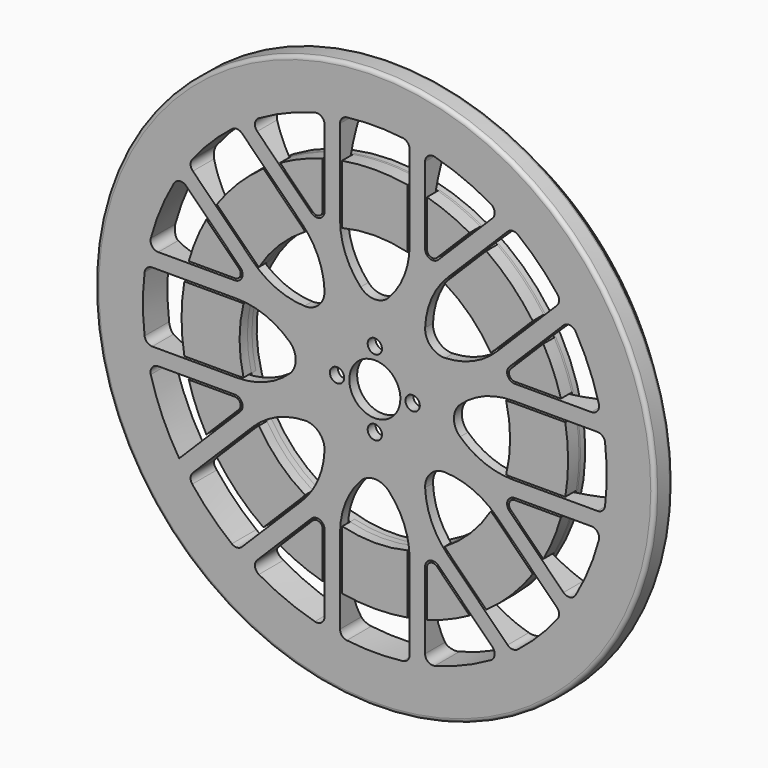
from build123d import *
from build123d import SkipClean  # not in build123d's __all__

# Parameters (mm, degrees)
F3_D      = 3.7
F4_R      = 71
F4_R_2    = 66
F4_R_3    = 6.604
F5_DEPTH  = 13.001
F6_R      = 20
F7_R      = 5
F8_R      = 2
F9_R      = 0.6
F13_DEPTH = 4
F14_R     = 72.39
F14_R_2   = 66
F15_DEPTH = 5.842
F16_R     = 1


with BuildPart() as f1:
    # F0 (on Right) → F1 (revolve)
    with BuildSketch(Plane.YZ):
        with BuildLine():
            Line((0, 66), (0, 6.604))
            Line((0, 6.604), (2.54, 6.604))
            Line((2.54, 6.604), (2.54, 42))
            ThreePointArc((2.54, 42), (5.2686233007, 55.0901833448), (13, 66))
            Line((13, 66), (0, 66))
        make_face()
    revolve(axis=Axis((0, 6.5, 0), (0, 1, 0)))

    # F3 (through all)
    with Locations(Plane.XZ):
        with Locations((0, 9.779), (9.779, 0), (0, -9.779), (-9.779, 0)):
            Hole(F3_D / 2)

    # F4 (on face) → F5 (cut, through all)
    with BuildSketch(Plane.XZ):
        Circle(F4_R)
        Circle(F4_R_2, mode=Mode.SUBTRACT)
        Circle(F4_R_3)
        with BuildLine():
            Line((-13, 25.7279220614), (-35.5824333316, 48.310355393))
            ThreePointArc((-35.5824333316, 48.310355393), (-42.4264068712, 42.4264068712), (-48.310355393, 35.5824333316))
            Line((-48.310355393, 35.5824333316), (-25.7279220614, 13))
            Line((-25.7279220614, 13), (-13, 13))
            Line((-13, 13), (-13, 25.7279220614))
        make_face()
        with BuildLine():
            ThreePointArc((-50.6109830133, 32.2262067024), (-55.4327719507, 22.9610059419), (-58.5747385824, 13))
            Line((-58.5747385824, 13), (-31.3847763109, 13))
            Line((-31.3847763109, 13), (-50.6109830133, 32.2262067024))
        make_face()
        with BuildLine():
            ThreePointArc((-59.3211597999, 9), (-60, 0), (-59.3211597999, -9))
            Line((-59.3211597999, -9), (-27.3847763109, -9))
            Line((-27.3847763109, -9), (-18.3847763109, 0))
            Line((-18.3847763109, 0), (-27.3847763109, 9))
            Line((-27.3847763109, 9), (-59.3211597999, 9))
        make_face()
        with BuildLine():
            Line((-31.3847763109, -13), (-58.5747385824, -13))
            ThreePointArc((-58.5747385824, -13), (-55.4327719507, -22.9610059419), (-50.6109830133, -32.2262067024))
            Line((-50.6109830133, -32.2262067024), (-31.3847763109, -13))
        make_face()
        with BuildLine():
            Line((-13, -25.7279220614), (-13, -13))
            Line((-13, -13), (-25.7279220614, -13))
            Line((-25.7279220614, -13), (-48.310355393, -35.5824333316))
            ThreePointArc((-48.310355393, -35.5824333316), (-42.4264068712, -42.4264068712), (-35.5824333316, -48.310355393))
            Line((-35.5824333316, -48.310355393), (-13, -25.7279220614))
        make_face()
        with BuildLine():
            Line((9, -27.3847763109), (0, -18.3847763109))
            Line((0, -18.3847763109), (-9, -27.3847763109))
            Line((-9, -27.3847763109), (-9, -59.3211597999))
            ThreePointArc((-9, -59.3211597999), (0, -60), (9, -59.3211597999))
            Line((9, -59.3211597999), (9, -27.3847763109))
        make_face()
        with BuildLine():
            Line((13, -31.3847763109), (13, -58.5747385824))
            ThreePointArc((13, -58.5747385824), (22.9610059419, -55.4327719507), (32.2262067024, -50.6109830133))
            Line((32.2262067024, -50.6109830133), (13, -31.3847763109))
        make_face()
        with BuildLine():
            Line((25.7279220614, -13), (13, -13))
            Line((13, -13), (13, -25.7279220614))
            Line((13, -25.7279220614), (35.5824333316, -48.310355393))
            ThreePointArc((35.5824333316, -48.310355393), (42.4264068712, -42.4264068712), (48.310355393, -35.5824333316))
            Line((48.310355393, -35.5824333316), (25.7279220614, -13))
        make_face()
        with BuildLine():
            Line((58.5747385824, -13), (31.3847763109, -13))
            Line((31.3847763109, -13), (50.6109830133, -32.2262067024))
            ThreePointArc((50.6109830133, -32.2262067024), (55.4327719507, -22.9610059419), (58.5747385824, -13))
        make_face()
        with BuildLine():
            Line((27.3847763109, 9), (18.3847763109, 0))
            Line((18.3847763109, 0), (27.3847763109, -9))
            Line((27.3847763109, -9), (59.3211597999, -9))
            ThreePointArc((59.3211597999, -9), (60, 0), (59.3211597999, 9))
            Line((59.3211597999, 9), (27.3847763109, 9))
        make_face()
        with BuildLine():
            Line((50.6109830133, 32.2262067024), (31.3847763109, 13))
            Line((31.3847763109, 13), (58.5747385824, 13))
            ThreePointArc((58.5747385824, 13), (55.4327719507, 22.9610059419), (50.6109830133, 32.2262067024))
        make_face()
        with BuildLine():
            Line((13, 25.7279220614), (13, 13))
            Line((13, 13), (25.7279220614, 13))
            Line((25.7279220614, 13), (48.310355393, 35.5824333316))
            ThreePointArc((48.310355393, 35.5824333316), (42.4264068712, 42.4264068712), (35.5824333316, 48.310355393))
            Line((35.5824333316, 48.310355393), (13, 25.7279220614))
        make_face()
        with BuildLine():
            Line((13, 58.5747385824), (13, 31.3847763109))
            Line((13, 31.3847763109), (32.2262067024, 50.6109830133))
            ThreePointArc((32.2262067024, 50.6109830133), (22.9610059419, 55.4327719507), (13, 58.5747385824))
        make_face()
        with BuildLine():
            Line((-9, 27.3847763109), (0, 18.3847763109))
            Line((0, 18.3847763109), (9, 27.3847763109))
            Line((9, 27.3847763109), (9, 59.3211597999))
            ThreePointArc((9, 59.3211597999), (0, 60), (-9, 59.3211597999))
            Line((-9, 59.3211597999), (-9, 27.3847763109))
        make_face()
        with BuildLine():
            Line((-13, 31.3847763109), (-13, 58.5747385824))
            ThreePointArc((-13, 58.5747385824), (-22.9610059419, 55.4327719507), (-32.2262067024, 50.6109830133))
            Line((-32.2262067024, 50.6109830133), (-13, 31.3847763109))
        make_face()
        with BuildLine():
            Line((-13, -31.3847763109), (-32.2262067024, -50.6109830133))
            ThreePointArc((-32.2262067024, -50.6109830133), (-22.9610059419, -55.4327719507), (-13, -58.5747385824))
            Line((-13, -58.5747385824), (-13, -31.3847763109))
        make_face()
    extrude(amount=-F5_DEPTH, mode=Mode.SUBTRACT)

    # F6
    f6_edges = [f1.edges().sort_by_distance(p)[0] for p in [
        (-9, 1.27, 27.384776),
        (9, 1.27, 27.384776),
        (13, 1.27, 25.727922),
        (25.727922, 1.27, 13),
        (27.384776, 1.27, 9),
        (27.384776, 1.27, -9),
        (25.727922, 1.27, -13),
        (9, 1.27, -27.384776),
        (13, 1.27, -25.727922),
        (-9, 1.27, -27.384776),
        (-13, 1.27, -25.727922),
        (-27.384776, 1.27, -9),
        (-25.727922, 1.27, -13),
        (-27.384776, 1.27, 9),
        (-13, 1.27, 25.727922),
        (-25.727922, 1.27, 13),
    ]]
    fillet(f6_edges, radius=F6_R)

    # F7
    f7_edges = [f1.edges().sort_by_distance(p)[0] for p in [
        (18.384776, 1.27, 0),
        (13, 1.27, 13),
        (0, 1.27, 18.384776),
        (-13, 1.27, 13),
        (-18.384776, 1.27, 0),
        (-13, 1.27, -13),
        (0, 1.27, -18.384776),
        (13, 1.27, -13),
    ]]
    fillet(f7_edges, radius=F7_R)

    # F8
    f8_edges = [f1.edges().sort_by_distance(p)[0] for p in [
        (-31.384776, 1.27, 13),
        (-13, 1.27, 31.384776),
        (13, 1.27, 31.384776),
        (31.384776, 1.27, 13),
        (31.384776, 1.27, -13),
        (13, 1.27, -31.384776),
        (-13, 1.27, -31.384776),
        (-31.384776, 1.27, -13),
        (-13, 3.96374, 58.574739),
        (-9, 3.96374, 59.32116),
        (-32.226207, 3.96374, 50.610983),
        (-35.582433, 3.96374, 48.310355),
        (-48.310355, 3.96374, 35.582433),
        (-50.610983, 3.96374, 32.226207),
        (-58.574739, 3.96374, 13),
        (-59.32116, 3.96374, -9),
        (-58.574739, 3.96374, -13),
        (-48.310355, 3.96374, -35.582433),
        (-59.32116, 3.96374, 9),
        (-35.582433, 3.96374, -48.310355),
        (-32.226207, 3.96374, -50.610983),
        (-9, 3.96374, -59.32116),
        (13, 3.96374, -58.574739),
        (-13, 3.96374, -58.574739),
        (9, 3.96374, -59.32116),
        (32.226207, 3.96374, -50.610983),
        (48.310355, 3.96374, -35.582433),
        (59.32116, 3.96374, -9),
        (35.582433, 3.96374, -48.310355),
        (50.610983, 3.96374, -32.226207),
        (58.574739, 3.96374, -13),
        (59.32116, 3.96374, 9),
        (58.574739, 3.96374, 13),
        (50.610983, 3.96374, 32.226207),
        (48.310355, 3.96374, 35.582433),
        (35.582433, 3.96374, 48.310355),
        (32.226207, 3.96374, 50.610983),
        (13, 3.96374, 58.574739),
        (9, 3.96374, 59.32116),
    ]]
    fillet(f8_edges, radius=F8_R)

    # F9
    f9_edges = [f1.edges().sort_by_distance(p)[0] for p in [
        (0, 13, -66),
    ]]
    fillet(f9_edges, radius=F9_R)

    # F14 (on face) → F15 (join)
    with BuildSketch(Plane.XZ):
        Circle(F14_R)
        Circle(F14_R_2, mode=Mode.SUBTRACT)
    extrude(amount=-F15_DEPTH)

    # F16
    f16_edges = [f1.edges().sort_by_distance(p)[0] for p in [
        (0, 5.842, -66),
        (-72.39, 0, 0),
        (-72.39, 5.842, 0),
    ]]
    fillet(f16_edges, radius=F16_R)


with BuildPart() as f11:
    # F10 (on Right) → F11 (revolve)
    with BuildSketch(Plane.YZ):
        with BuildLine():
            Line((5.54, 50), (3.5317066212, 50))
            ThreePointArc((3.5317066212, 50), (2.788871873, 46.0306166409), (2.54, 42))
            Line((2.54, 42), (2.54, 35))
            Line((2.54, 35), (5.54, 35))
            Line((5.54, 35), (5.54, 50))
        make_face()
    revolve(axis=Axis((0, 2.77, 0), (0, 1, 0)))

    # F12 (on face) → F13 (join)
    with BuildSketch(Plane.XZ):
        with BuildLine():
            ThreePointArc((-29.9788766201, 18.0628612517), (-24.7487373415, 24.7487373415), (-18.0628612517, 29.9788766201))
            ThreePointArc((-18.0628612517, 29.9788766201), (-18.6234744441, 30.6180772887), (-19.2114177669, 31.232233047))
            Line((-19.2114177669, 31.232233047), (-28.8303013079, 40.8511165881))
            ThreePointArc((-28.8303013079, 40.8511165881), (-35.3553390593, 35.3553390593), (-40.8511165881, 28.8303013079))
            Line((-40.8511165881, 28.8303013079), (-31.232233047, 19.2114177669))
            ThreePointArc((-31.232233047, 19.2114177669), (-30.6180772887, 18.6234744441), (-29.9788766201, 18.0628612517))
        make_face()
        with BuildLine():
            Line((-13.5, 36.2132034356), (-13.5, 48.1430161083))
            ThreePointArc((-13.5, 48.1430161083), (-19.1341716183, 46.1939766256), (-24.4963116109, 43.5881947029))
            Line((-24.4963116109, 43.5881947029), (-16.0606601718, 35.1525432638))
            ThreePointArc((-16.0606601718, 35.1525432638), (-14.4259748515, 34.8273841368), (-13.5, 36.2132034356))
        make_face()
        with BuildLine():
            Line((-35.6690475583, 8.5), (-49.272203117, 8.5))
            ThreePointArc((-49.272203117, 8.5), (-50, 0), (-49.272203117, -8.5))
            Line((-49.272203117, -8.5), (-35.6690475583, -8.5))
            ThreePointArc((-35.6690475583, -8.5), (-34.8190351464, -8.4814650091), (-33.9706386291, -8.4258952718))
            ThreePointArc((-33.9706386291, -8.4258952718), (-35, 0), (-33.9706386291, 8.4258952718))
            ThreePointArc((-33.9706386291, 8.4258952718), (-34.8190351464, 8.4814650091), (-35.6690475583, 8.5))
        make_face()
        with BuildLine():
            ThreePointArc((-43.5881947029, 24.4963116109), (-46.1939766256, 19.1341716183), (-48.1430161083, 13.5))
            Line((-48.1430161083, 13.5), (-36.2132034356, 13.5))
            ThreePointArc((-36.2132034356, 13.5), (-34.8273841368, 14.4259748515), (-35.1525432638, 16.0606601718))
            Line((-35.1525432638, 16.0606601718), (-43.5881947029, 24.4963116109))
        make_face()
        with BuildLine():
            Line((-31.232233047, -19.2114177669), (-40.8511165881, -28.8303013079))
            ThreePointArc((-40.8511165881, -28.8303013079), (-35.3553390593, -35.3553390593), (-28.8303013079, -40.8511165881))
            Line((-28.8303013079, -40.8511165881), (-19.2114177669, -31.232233047))
            ThreePointArc((-19.2114177669, -31.232233047), (-18.6234744441, -30.6180772887), (-18.0628612517, -29.9788766201))
            ThreePointArc((-18.0628612517, -29.9788766201), (-24.7487373415, -24.7487373415), (-29.9788766201, -18.0628612517))
            ThreePointArc((-29.9788766201, -18.0628612517), (-30.6180772887, -18.6234744441), (-31.232233047, -19.2114177669))
        make_face()
        with BuildLine():
            ThreePointArc((-48.1430161083, -13.5), (-46.1939766256, -19.1341716183), (-43.5881947029, -24.4963116109))
            Line((-43.5881947029, -24.4963116109), (-35.1525432638, -16.0606601718))
            ThreePointArc((-35.1525432638, -16.0606601718), (-34.8273841368, -14.4259748515), (-36.2132034356, -13.5))
            Line((-36.2132034356, -13.5), (-48.1430161083, -13.5))
        make_face()
        with BuildLine():
            Line((-8.5, -35.6690475583), (-8.5, -49.272203117))
            ThreePointArc((-8.5, -49.272203117), (0, -50), (8.5, -49.272203117))
            Line((8.5, -49.272203117), (8.5, -35.6690475583))
            ThreePointArc((8.5, -35.6690475583), (8.4814650091, -34.8190351464), (8.4258952718, -33.9706386291))
            ThreePointArc((8.4258952718, -33.9706386291), (0, -35), (-8.4258952718, -33.9706386291))
            ThreePointArc((-8.4258952718, -33.9706386291), (-8.4814650091, -34.8190351464), (-8.5, -35.6690475583))
        make_face()
        with BuildLine():
            ThreePointArc((-24.4963116109, -43.5881947029), (-19.1341716183, -46.1939766256), (-13.5, -48.1430161083))
            Line((-13.5, -48.1430161083), (-13.5, -36.2132034356))
            ThreePointArc((-13.5, -36.2132034356), (-14.4259748515, -34.8273841368), (-16.0606601718, -35.1525432638))
            Line((-16.0606601718, -35.1525432638), (-24.4963116109, -43.5881947029))
        make_face()
        with BuildLine():
            Line((19.2114177669, -31.232233047), (28.8303013079, -40.8511165881))
            ThreePointArc((28.8303013079, -40.8511165881), (35.3553390593, -35.3553390593), (40.8511165881, -28.8303013079))
            Line((40.8511165881, -28.8303013079), (31.232233047, -19.2114177669))
            ThreePointArc((31.232233047, -19.2114177669), (30.6180772887, -18.6234744441), (29.9788766201, -18.0628612517))
            ThreePointArc((29.9788766201, -18.0628612517), (24.7487373415, -24.7487373415), (18.0628612517, -29.9788766201))
            ThreePointArc((18.0628612517, -29.9788766201), (18.6234744441, -30.6180772887), (19.2114177669, -31.232233047))
        make_face()
        with BuildLine():
            ThreePointArc((13.5, -48.1430161083), (19.1341716183, -46.1939766256), (24.4963116109, -43.5881947029))
            Line((24.4963116109, -43.5881947029), (16.0606601718, -35.1525432638))
            ThreePointArc((16.0606601718, -35.1525432638), (14.4259748515, -34.8273841368), (13.5, -36.2132034356))
            Line((13.5, -36.2132034356), (13.5, -48.1430161083))
        make_face()
        with BuildLine():
            Line((35.6690475583, -8.5), (49.272203117, -8.5))
            ThreePointArc((49.272203117, -8.5), (50, 0), (49.272203117, 8.5))
            Line((49.272203117, 8.5), (35.6690475583, 8.5))
            ThreePointArc((35.6690475583, 8.5), (34.8190351464, 8.4814650091), (33.9706386291, 8.4258952718))
            ThreePointArc((33.9706386291, 8.4258952718), (35, 0), (33.9706386291, -8.4258952718))
            ThreePointArc((33.9706386291, -8.4258952718), (34.8190351464, -8.4814650091), (35.6690475583, -8.5))
        make_face()
        with BuildLine():
            ThreePointArc((43.5881947029, -24.4963116109), (46.1939766256, -19.1341716183), (48.1430161083, -13.5))
            Line((48.1430161083, -13.5), (36.2132034356, -13.5))
            ThreePointArc((36.2132034356, -13.5), (34.8273841368, -14.4259748515), (35.1525432638, -16.0606601718))
            Line((35.1525432638, -16.0606601718), (43.5881947029, -24.4963116109))
        make_face()
        with BuildLine():
            Line((31.232233047, 19.2114177669), (40.8511165881, 28.8303013079))
            ThreePointArc((40.8511165881, 28.8303013079), (35.3553390593, 35.3553390593), (28.8303013079, 40.8511165881))
            Line((28.8303013079, 40.8511165881), (19.2114177669, 31.232233047))
            ThreePointArc((19.2114177669, 31.232233047), (18.6234744441, 30.6180772887), (18.0628612517, 29.9788766201))
            ThreePointArc((18.0628612517, 29.9788766201), (24.7487373415, 24.7487373415), (29.9788766201, 18.0628612517))
            ThreePointArc((29.9788766201, 18.0628612517), (30.6180772887, 18.6234744441), (31.232233047, 19.2114177669))
        make_face()
        with BuildLine():
            ThreePointArc((48.1430161083, 13.5), (46.1939766256, 19.1341716183), (43.5881947029, 24.4963116109))
            Line((43.5881947029, 24.4963116109), (35.1525432638, 16.0606601718))
            ThreePointArc((35.1525432638, 16.0606601718), (34.8273841368, 14.4259748515), (36.2132034356, 13.5))
            Line((36.2132034356, 13.5), (48.1430161083, 13.5))
        make_face()
        with BuildLine():
            Line((8.5, 35.6690475583), (8.5, 49.272203117))
            ThreePointArc((8.5, 49.272203117), (0, 50), (-8.5, 49.272203117))
            Line((-8.5, 49.272203117), (-8.5, 35.6690475583))
            ThreePointArc((-8.5, 35.6690475583), (-8.4814650091, 34.8190351464), (-8.4258952718, 33.9706386291))
            ThreePointArc((-8.4258952718, 33.9706386291), (0, 35), (8.4258952718, 33.9706386291))
            ThreePointArc((8.4258952718, 33.9706386291), (8.4814650091, 34.8190351464), (8.5, 35.6690475583))
        make_face()
        with BuildLine():
            ThreePointArc((24.4963116109, 43.5881947029), (19.1341716183, 46.1939766256), (13.5, 48.1430161083))
            Line((13.5, 48.1430161083), (13.5, 36.2132034356))
            ThreePointArc((13.5, 36.2132034356), (14.4259748515, 34.8273841368), (16.0606601718, 35.1525432638))
            Line((16.0606601718, 35.1525432638), (24.4963116109, 43.5881947029))
        make_face()
    with SkipClean():  # cleaning this boolean's faces spoils the solid; the shape is the same uncleaned
        extrude(amount=-F13_DEPTH)


solid = Compound([f1.part, f11.part])
